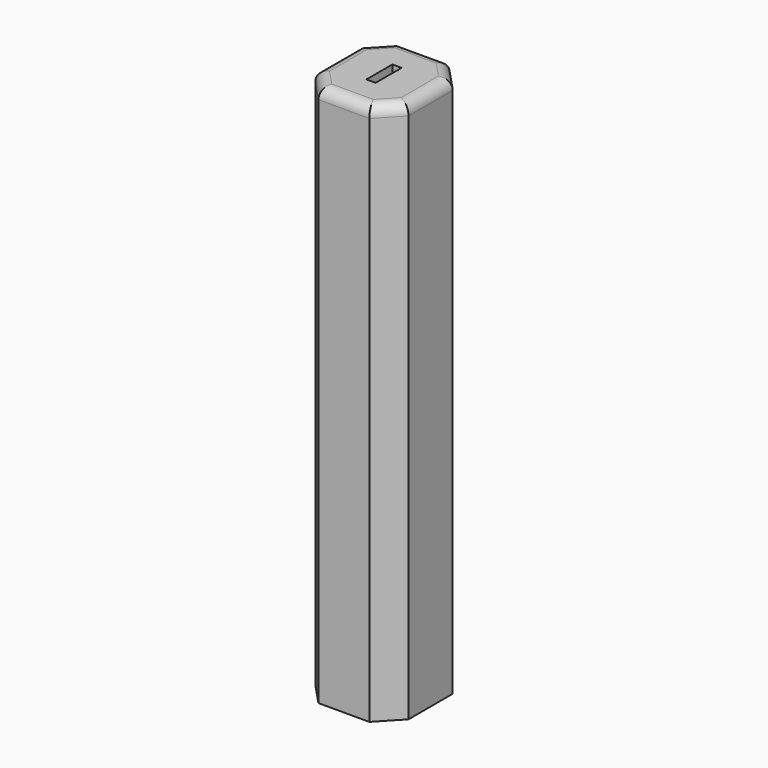
from build123d import *

# Parameters (mm, degrees)
F1_DEPTH    = 127
F2_W        = 2.159
F2_H        = 7.62
F3_DEPTH    = 63.5
F4_T        = -2.54
F5_R        = 2.54
F6_T4_DEPTH = 20.1763121576


# Not quite as in the source:
# - a fillet or chamfer that OpenCascade refuses, or shapes differently, is made with other operations: its cross-section is extruded or revolved along the edge and cut away or added


with BuildPart() as f1:
    # F0 (on Top) → F1 (new body)
    with BuildSketch(Plane.XY):
        Polygon((-5.969, -11.7475), (5.969, -11.7475), (10.922, -6.477), (10.922, 6.477), (5.969, 11.7475), (-5.969, 11.7475), (-10.922, 6.477), (-10.922, -6.477), align=None)
    extrude(amount=F1_DEPTH)

    # F2 (on face) → F3 (cut)
    with BuildSketch(Plane.XY.offset(127)):
        Rectangle(F2_W, F2_H)
    extrude(amount=-F3_DEPTH, mode=Mode.SUBTRACT)

    # F4
    f4_openings = [f1.faces().sort_by_distance(p)[0] for p in [
        (0, 0, 0),
    ]]
    offset(amount=F4_T, openings=f4_openings, kind=Kind.INTERSECTION)

    # F5
    f5_edges = [f1.edges().sort_by_distance(p)[0] for p in [
        (10.922, 0, 127),
        (0, 11.7475, 127),
        (-10.922, 0, 127),
        (0, -11.7475, 127),
        (-8.4455, 9.11225, 127),
        (8.4455, 9.11225, 127),
        (8.4455, -9.11225, 127),
        (-8.4455, -9.11225, 127),
    ]]
    fillet(f5_edges, radius=F5_R)

    # F6: fillet of radius 2.54 on 1 edges, made by hand


with BuildPart() as f6_tool2:
    # F6_s3 → F6_t4 (new body)
    with BuildSketch(Plane.XZ.offset(10.0881560788)):
        with BuildLine():
            ThreePointArc((1.0795, 66.0112624315), (0.4655503628, 64.3553850206), (-1.0795, 63.5))
            Line((-1.0795, 63.5), (1.0795, 63.5))
            Line((1.0795, 63.5), (1.0795, 66.0112624315))
        make_face()
    extrude(amount=-F6_T4_DEPTH)

    split(bisect_by=Plane.XZ.offset(6.35), keep=Keep.BOTTOM)

    split(bisect_by=Plane.XZ.offset(-6.35), keep=Keep.TOP)


with BuildPart() as f1_1:
    add(f1.part)

    # F6_t1: union F6_tool2
    add(f6_tool2.part)


solid = f1_1.part
